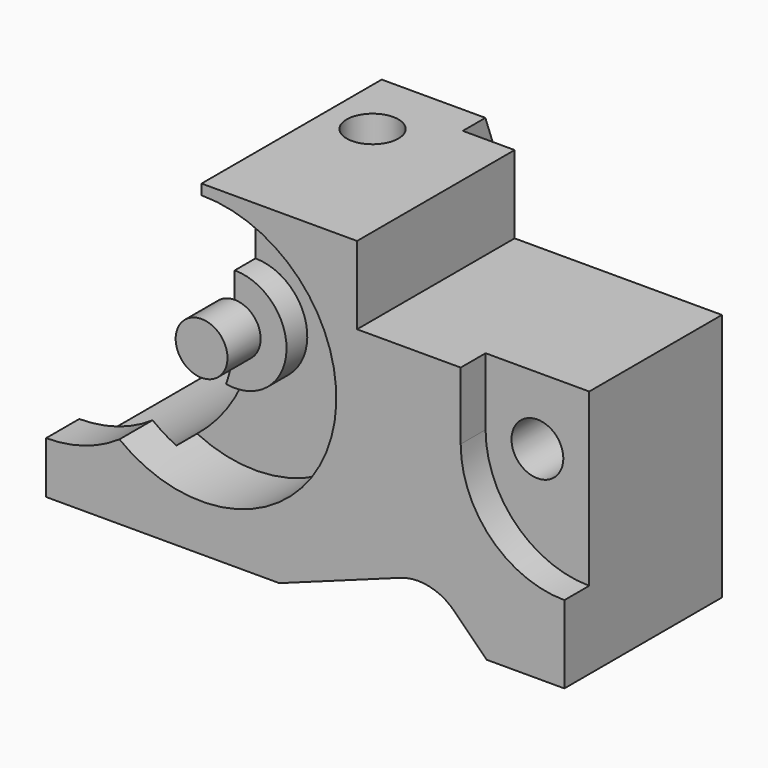
from build123d import *

# Parameters (mm, degrees)
F0_W      = 100
F0_H      = 63
F1_DEPTH  = 50
F2_W      = 40
F2_H      = 15
F3_DEPTH  = 50.001
F4_R      = 5
F5_DEPTH  = 50.001
F7_DEPTH  = 50.001
F9_DEPTH  = 6
F10_W     = 50
F10_H     = 12
F11_DEPTH = 63.001
F12_R     = 26
F12_R_2   = 10
F13_DEPTH = 13
F14_R     = 10
F14_R_2   = 5
F15_DEPTH = 8
F17_DEPTH = 8
F19_DEPTH = 42
F21_DEPTH = 70.001
F22_R     = 5
F23_DEPTH = 63.001


with BuildPart() as f1:
    # F0 (on Front) → F1 (new body)
    with BuildSketch(Plane.XZ):
        with Locations((50, 31.5)):
            Rectangle(F0_W, F0_H)
    extrude(amount=F1_DEPTH)

    # F2 (on face) → F3 (cut, through all)
    with BuildSketch(Plane.XZ.offset(50)):
        with Locations((80, 55.5)):
            Rectangle(F2_W, F2_H)
    extrude(amount=-F3_DEPTH, mode=Mode.SUBTRACT)

    # F4 (on face) → F5 (cut, through all)
    with BuildSketch(Plane.XZ.offset(50)):
        with Locations((90, 35)):
            Circle(F4_R)
    extrude(amount=-F5_DEPTH, mode=Mode.SUBTRACT)

    # F6 (on face) → F7 (cut, through all)
    with BuildSketch(Plane.XZ.offset(50)):
        with BuildLine():
            Line((68.3396509331, 8.4949382178), (45, 0))
            Line((45, 0), (85, 0))
            Line((85, 0), (78.8309201782, 6.1690798218))
            ThreePointArc((78.8309201782, 6.1690798218), (73.9242485057, 8.8609720811), (68.3396509331, 8.4949382178))
        make_face()
    extrude(amount=-F7_DEPTH, mode=Mode.SUBTRACT)

    # F8 (on face) → F9 (cut)
    with BuildSketch(Plane.XZ.offset(50)):
        with BuildLine():
            Line((100, 48), (80, 48))
            Line((80, 48), (80, 35))
            ThreePointArc((80, 35), (85.8578643763, 20.8578643763), (100, 15))
            Line((100, 15), (100, 48))
        make_face()
    extrude(amount=-F9_DEPTH, mode=Mode.SUBTRACT)

    # F10 (on face) → F11 (cut, through all)
    with BuildSketch(Plane.XY.offset(63)):
        with Locations((75, -6)):
            Rectangle(F10_W, F10_H)
    extrude(amount=-F11_DEPTH, mode=Mode.SUBTRACT)

    # F12 (on face) → F13 (cut)
    with BuildSketch(Plane.XZ.offset(50)):
        with Locations((30, 35)):
            Circle(F12_R)
        with Locations((30, 35)):
            Circle(F12_R_2, mode=Mode.SUBTRACT)
    extrude(amount=-F13_DEPTH, mode=Mode.SUBTRACT)

    # F14 (on face) → F15 (cut)
    with BuildSketch(Plane.XZ.offset(50)):
        with Locations((30, 35)):
            Circle(F14_R)
        with Locations((30, 35)):
            Circle(F14_R_2, mode=Mode.SUBTRACT)
    extrude(amount=-F15_DEPTH, mode=Mode.SUBTRACT)

    # F16 (on face) → F17 (cut)
    with BuildSketch(Plane.XZ.offset(50)):
        with BuildLine():
            Line((0, 35), (0, 10))
            ThreePointArc((0, 10), (7.407655665, 11.122675243), (14.15, 14.389868996))
            ThreePointArc((14.15, 14.389868996), (5.3843199758, 43.3706807936), (30, 61))
            Line((30, 61), (30, 63))
            Line((30, 63), (0, 63))
            Line((0, 63), (0, 35))
        make_face()
    extrude(amount=-F17_DEPTH, mode=Mode.SUBTRACT)

    # F18 (on face) → F19 (cut, through all)
    with BuildSketch(Plane(origin=(0, 0, 0), x_dir=(-1, 0, 0), z_dir=(0, 1, 0))):
        with BuildLine():
            Line((-30, 63), (-30, 35))
            ThreePointArc((-30, 35), (-21.2132034356, 13.7867965644), (0, 5))
            Line((0, 5), (0, 63))
            Line((0, 63), (-30, 63))
        make_face()
    extrude(amount=-F19_DEPTH, mode=Mode.SUBTRACT)

    # F20 (on face) → F21 (cut, through all)
    with BuildSketch(Plane(origin=(30, 0, 0), x_dir=(0, -1, 0), z_dir=(-1, 0, 0))):
        Polygon((0, 45), (6.5514642168, 63), (0, 63), align=None)
    extrude(amount=-F21_DEPTH, mode=Mode.SUBTRACT)

    # F22 (on face) → F23 (cut, through all)
    with BuildSketch(Plane.XY.offset(63)):
        with Locations((39, -20)):
            Circle(F22_R)
    extrude(amount=-F23_DEPTH, mode=Mode.SUBTRACT)


solid = f1.part
